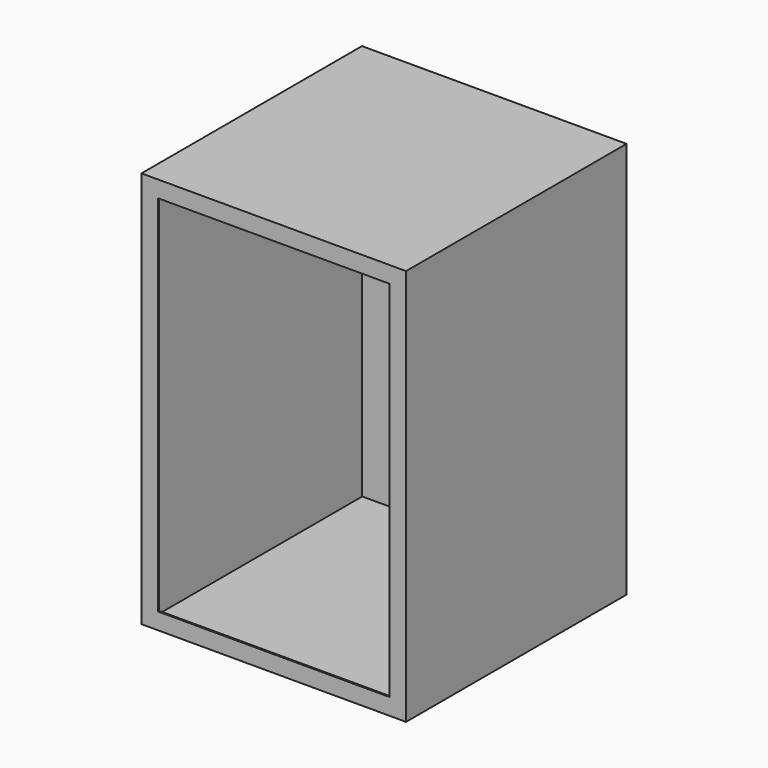
from build123d import *

# Parameters (mm, degrees)
F0_W     = 609.6
F0_H     = 914.4
F1_DEPTH = 609.6
F2_DEPTH = 25.4
F3_T     = -3.302
F4_W     = 533.4
F4_H     = 838.2
F5_DEPTH = 584.2


with BuildPart() as f1:
    # F0 (on Front) → F1 (new body)
    with BuildSketch(Plane.XZ):
        with Locations((-127.1454390585, -4.6617306446)):
            Rectangle(F0_W, F0_H)
    extrude(amount=F1_DEPTH)

    # F2 (add): a face of the model
    f2_faces = [f1.faces().sort_by_distance(p)[0] for p in [
        (-127.1454390585, -609.6, -4.6617306446),
    ]]
    extrude(f2_faces, amount=F2_DEPTH)

    # F3 (hollow: no face is removed)
    offset(amount=F3_T, mode=Mode.SUBTRACT)

    # F4 (on face) → F5 (cut)
    with BuildSketch(Plane.XZ.offset(635)):
        with Locations((-127.1454390585, -4.6617306446)):
            Rectangle(F4_W, F4_H)
    extrude(amount=-F5_DEPTH, mode=Mode.SUBTRACT)


solid = f1.part
